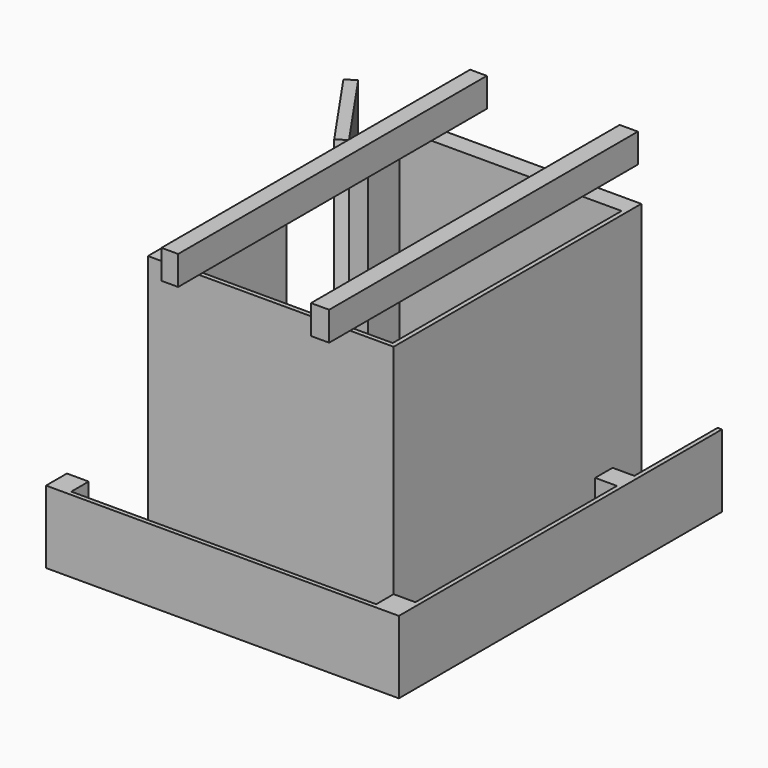
from build123d import *

# Parameters (mm, degrees)
F0_W     = 100
F0_H     = 40
F0_W_2   = 130
F0_H_2   = 65.0866451263
F1_DEPTH = 1040
F0_W_3   = 50
F0_H_3   = 25
F2_DEPTH = 1040
F3_DEPTH = 1041
F4_DEPTH = 1050
F0_W_4   = 31
F0_H_4   = 131
F0_H_5   = 31
F5_DEPTH = 2000
F6_W     = 125
F6_H     = 2657.3488712311
F6_W_2   = 115
F7_DEPTH = 200
F0_W_5   = 150
F0_H_6   = 150
F8_DEPTH = 500


# Not quite as in the source:
# - a feature names something its author has since deleted; it is built from what else it names


with BuildPart() as f1:
    # F0 (on Top) → F1 (new body)
    with BuildSketch(Plane.XY):
        with BuildLine():
            ThreePointArc((-845.2893218813, 1881), (-916, 1861), (-986.7106781187, 1881))
            Line((-986.7106781187, 1881), (-1141, 1881))
            Line((-1141, 1881), (-1141, 1161.5))
            ThreePointArc((-1141, 1161.5), (-1140.6464466094, 1161.3535533906), (-1140.5, 1161))
            ThreePointArc((-1140.5, 1161), (-1140.5380602337, 1160.8086582838), (-1140.6464466094, 1160.6464466094))
            Line((-1140.6464466094, 1160.6464466094), (-1091, 1111))
            Line((-1091, 1111), (-741, 1111))
            Line((-741, 1111), (-691, 1161))
            Line((-691, 1161), (-691, 1881))
            Line((-691, 1881), (-845.2893218813, 1881))
        make_face()
        with Locations((-916, 1201)):
            Rectangle(F0_W, F0_H, mode=Mode.SUBTRACT)
        with BuildLine():
            Line((-851, 1881), (-981, 1881))
            Line((-981, 1881), (-986.7106781187, 1881))
            ThreePointArc((-986.7106781187, 1881), (-916, 1861), (-845.2893218813, 1881))
            Line((-845.2893218813, 1881), (-851, 1881))
        make_face()
        with BuildLine():
            Line((-1141.2869326556, 1160.590525152), (-1141, 1161))
            Line((-1141, 1161), (-1141.4924344683, 1160.9133495848))
            ThreePointArc((-1141.4924344683, 1160.9133495848), (-1141.421790448, 1160.7314989424), (-1141.2869326556, 1160.590525152))
        make_face()
        with BuildLine():
            ThreePointArc((-1141.2869326556, 1160.590525152), (-1141.421790448, 1160.7314989424), (-1141.4924344683, 1160.9133495848))
            Line((-1141.4924344683, 1160.9133495848), (-1210.6407503609, 1148.7457807602))
            Line((-1210.6407503609, 1148.7457807602), (-1411.4936092846, 862.1133871579))
            Line((-1411.4936092846, 862.1133871579), (-1399.2393900448, 792.4726367971))
            Line((-1399.2393900448, 792.4726367971), (-1141.2869326556, 1160.590525152))
        make_face()
        with BuildLine():
            ThreePointArc((-1140.5, 1161), (-1140.6464466094, 1161.3535533906), (-1141, 1161.5))
            Line((-1141, 1161.5), (-1141, 1161))
            Line((-1141, 1161), (-1140.6464466094, 1160.6464466094))
            ThreePointArc((-1140.6464466094, 1160.6464466094), (-1140.5380602337, 1160.8086582838), (-1140.5, 1161))
        make_face()
        with BuildLine():
            Line((-1140.6464466094, 1160.6464466094), (-1141, 1161))
            Line((-1141, 1161), (-1141.2869326556, 1160.590525152))
            ThreePointArc((-1141.2869326556, 1160.590525152), (-1140.9565099674, 1160.5018949739), (-1140.6464466094, 1160.6464466094))
        make_face()
        with BuildLine():
            Line((-1141, 1161), (-1141, 1161.5))
            ThreePointArc((-1141, 1161.5), (-1141.3829655387, 1161.3214613448), (-1141.4924344683, 1160.9133495848))
            Line((-1141.4924344683, 1160.9133495848), (-1141, 1161))
        make_face()
        with Locations((-916, 1913.5433225632)):
            Rectangle(F0_W_2, F0_H_2)
        with BuildLine():
            Line((-986.7106781187, 1881), (-981, 1881))
            Line((-981, 1881), (-981, 1946.0866451263))
            Line((-981, 1946.0866451263), (-851, 1946.0866451263))
            Line((-851, 1946.0866451263), (-851, 1881))
            Line((-851, 1881), (-845.2893218813, 1881))
            ThreePointArc((-845.2893218813, 1881), (-798.1633725321, 1930.1248967592), (-781, 1996))
            ThreePointArc((-781, 1996), (-981.8751032408, 2113.8366274679), (-986.7106781187, 1881))
        make_face()
    extrude(amount=F1_DEPTH)


with BuildPart() as f2:
    # F0 (on Top) → F2 (new body)
    with BuildSketch(Plane.XY):
        Polygon((-691, 2131), (-691, 1881), (-691, 1161), (-641, 1111), (-281, 1111), (-231, 1161), (-231, 2131), align=None)
        Polygon((-656, 1361), (-656, 1871), (-591, 1871), (-591, 1896), (-541, 1896), (-541, 1871), (-381, 1871), (-381, 1896), (-331, 1896), (-331, 1871), (-266, 1871), (-266, 1361), align=None, mode=Mode.SUBTRACT)
        Polygon((-591, 1871), (-656, 1871), (-656, 1361), (-266, 1361), (-266, 1871), (-331, 1871), (-331, 1846), (-381, 1846), (-381, 1871), (-541, 1871), (-541, 1846), (-591, 1846), align=None)
        with Locations((-461, 1451)):
            Rectangle(F0_W, F0_H, mode=Mode.SUBTRACT)
        with Locations((-461, 1451)):
            Rectangle(F0_W, F0_H)
        with Locations((-566, 1858.5)):
            Rectangle(F0_W_3, F0_H_3)
        with Locations((-566, 1883.5)):
            Rectangle(F0_W_3, F0_H_3)
        with Locations((-356, 1883.5)):
            Rectangle(F0_W_3, F0_H_3)
        with Locations((-356, 1858.5)):
            Rectangle(F0_W_3, F0_H_3)
    extrude(amount=F2_DEPTH)

    # F0 (on Top) → F3 (join)
    with BuildSketch(Plane.XY):
        Polygon((-591, 1871), (-656, 1871), (-656, 1361), (-266, 1361), (-266, 1871), (-331, 1871), (-331, 1846), (-381, 1846), (-381, 1871), (-541, 1871), (-541, 1846), (-591, 1846), align=None)
        with Locations((-461, 1451)):
            Rectangle(F0_W, F0_H, mode=Mode.SUBTRACT)
    extrude(amount=F3_DEPTH)

    # F0 (on Top) → F4 (join)
    with BuildSketch(Plane.XY):
        with Locations((-566, 1883.5)):
            Rectangle(F0_W_3, F0_H_3)
        with Locations((-566, 1858.5)):
            Rectangle(F0_W_3, F0_H_3)
        with Locations((-356, 1883.5)):
            Rectangle(F0_W_3, F0_H_3)
        with Locations((-356, 1858.5)):
            Rectangle(F0_W_3, F0_H_3)
    extrude(amount=F4_DEPTH)


with BuildPart() as f5:
    # F0 (on Top) → F5 (new body)
    with BuildSketch(Plane.XY):
        with BuildLine():
            Line((-1741, 2181), (-211, 2181))
            Line((-211, 2181), (-211, 2312))
            Line((-211, 2312), (-1872, 2312))
            Line((-1872, 2312), (-1872, 1911.4519278278))
            ThreePointArc((-1872, 1911.4519278278), (-1871.6804387684, 1911.3195612316), (-1871.5480721722, 1911))
            Line((-1871.5480721722, 1911), (-1741, 1911))
            Line((-1741, 1911), (-1741, 2181))
        make_face()
        with Locations((-195.5, 2246.5)):
            Rectangle(F0_W_4, F0_H_4)
        Polygon((-180, 1915.0275195633), (-180, 2065.0275195633), (-180, 2181), (-211, 2181), (-211, 211), (-180, 211), align=None)
        with Locations((-195.5, 195.5)):
            Rectangle(F0_W_4, F0_H_5)
        Polygon((-1872, 180), (-211, 180), (-211, 211), (-1741, 211), (-1741, 1211), (-1872, 1211), align=None)
        with BuildLine():
            Line((-1872.3719540131, 1910.743311524), (-1872, 1911))
            Line((-1872, 1911), (-1872.256688476, 1911.3719540131))
            ThreePointArc((-1872.256688476, 1911.3719540131), (-1872.444517367, 1911.0815050429), (-1872.3719540131, 1910.743311524))
        make_face()
        with BuildLine():
            ThreePointArc((-1872.3719540131, 1910.743311524), (-1872.444517367, 1911.0815050429), (-1872.256688476, 1911.3719540131))
            Line((-1872.256688476, 1911.3719540131), (-2269.5898852459, 2487.1269679074))
            Line((-2269.5898852459, 2487.1269679074), (-2335.4329672925, 2441.6881238793))
            Line((-2335.4329672925, 2441.6881238793), (-1937.8430820466, 1865.5611559719))
            Line((-1937.8430820466, 1865.5611559719), (-1872.3719540131, 1910.743311524))
        make_face()
        with BuildLine():
            ThreePointArc((-1871.5480721722, 1911), (-1871.6804387684, 1911.3195612316), (-1872, 1911.4519278278))
            Line((-1872, 1911.4519278278), (-1872, 1911))
            Line((-1872, 1911), (-1871.5480721722, 1911))
        make_face()
        with BuildLine():
            Line((-1872, 1911), (-1872, 1911.4519278278))
            ThreePointArc((-1872, 1911.4519278278), (-1872.1344291493, 1911.4314713958), (-1872.256688476, 1911.3719540131))
            Line((-1872.256688476, 1911.3719540131), (-1872, 1911))
        make_face()
    extrude(amount=F5_DEPTH)

    # F6 (on face) → F7 (join)
    with BuildSketch(Plane.XY.offset(2000)):
        with Locations((-542.5, 1328.6744356155)):
            Rectangle(F6_W, F6_H)
        with Locations((-1577.5, 1328.6744356155)):
            Rectangle(F6_W_2, F6_H)
    extrude(amount=F7_DEPTH)


with BuildPart() as f8:
    # F0 (on Top) → F8 (new body)
    with BuildSketch(Plane.XY):
        with Locations((-2355, 105)):
            Rectangle(F0_W_5, F0_H_6)
        with BuildLine():
            Line((0, 2781.2819480896), (-30, 2781.2819480896))
            Line((-30, 2781.2819480896), (-30, 2065.0275195633))
            Line((-30, 2065.0275195633), (-30, 1915.0275195633))
            Line((-30, 1915.0275195633), (-30, 180))
            Line((-30, 180), (-30, 30))
            Line((-30, 30), (-180, 30))
            Line((-180, 30), (-2280, 30))
            Line((-2280, 30), (-2430, 30))
            Line((-2430, 30), (-2430, 0.5))
            ThreePointArc((-2430, 0.5), (-2429.6464466094, 0.3535533906), (-2429.5, 0))
            Line((-2429.5, 0), (0, 0))
            Line((0, 0), (0, 2781.2819480896))
        make_face()
        with Locations((-105, 105)):
            Rectangle(F0_W_5, F0_H_6)
        with Locations((-105, 1990.0275195633)):
            Rectangle(F0_W_5, F0_H_6)
    extrude(amount=F8_DEPTH)


solid = Compound([f1.part, f2.part, f5.part, f8.part])
